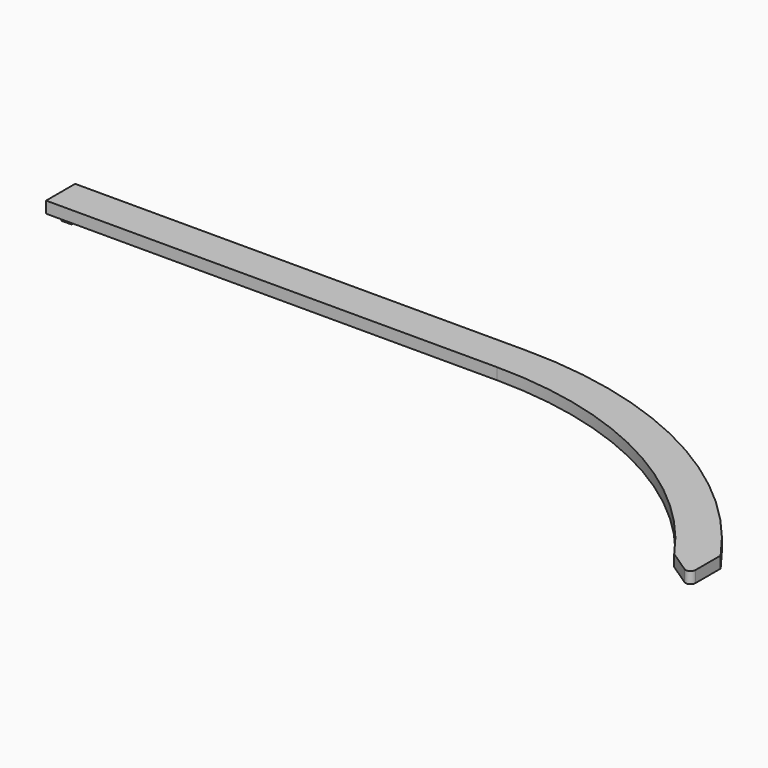
from build123d import *

# Parameters (mm, degrees)
F1_DEPTH = 2.3
F3_DEPTH = 2


with BuildPart() as f1:
    # F0 (on Top) → F1 (new body)
    with BuildSketch(Plane.XY):
        Polygon((45, 3.625), (-45, 3.625), (-45, 0), (-45, -3.625), (45, -3.625), align=None)
        Polygon((-44, -1), (-44, 0), (-44, 1), (-42, 1), (-42, -1), align=None, mode=Mode.SUBTRACT)
        with BuildLine():
            ThreePointArc((111.9139716029, -31.496938318), (82.7856789898, -5.6889854515), (45, 3.625))
            Line((45, 3.625), (45, -3.625))
            ThreePointArc((45, -3.625), (79.4162271285, -12.1084320129), (105.947070592, -35.615019464))
            Line((105.947070592, -35.615019464), (110.3610228539, -38.574432601))
            ThreePointArc((110.3610228539, -38.574432601), (111.3860089549, -38.6260052928), (111.9139716029, -37.7459418336))
            Line((111.9139716029, -37.7459418336), (111.9139716029, -31.496938318))
        make_face()
        Polygon((-44, 1), (-44, 0), (-44, -1), (-42, -1), (-42, 1), align=None)
    extrude(amount=-F1_DEPTH)

    # F2 (on face) → F3 (join)
    with BuildSketch(Plane(origin=(0, 0, -2.3), x_dir=(1, 0, 0), z_dir=(0, 0, -1))):
        Polygon((-44, 1), (-44, 0), (-44, -1), (-42, -1), (-42, 1), align=None)
    extrude(amount=F3_DEPTH)

    # F6 (on face) → F7 (revolve)
    with BuildSketch(Plane(origin=(0, 1, 0), x_dir=(-1, 0, 0), z_dir=(0, 1, 0))):
        with BuildLine():
            ThreePointArc((43.5, -3.3), (43.3535533906, -2.9464466094), (43, -2.8))
            Line((43, -2.8), (43, -3.3))
            Line((43, -3.3), (43.5, -3.3))
        make_face()
        with BuildLine():
            Line((43.5, -3.3), (43, -3.3))
            Line((43, -3.3), (43, -3.8))
            ThreePointArc((43, -3.8), (43.3535533906, -3.6535533906), (43.5, -3.3))
        make_face()
    revolve(axis=Axis((-43, 1, -3.3), (0, 0, -1)))


with BuildPart() as f5:
    # F4 (on face) → F5 (revolve)
    with BuildSketch(Plane.XZ.offset(1)):
        with BuildLine():
            Line((-43, -3.3), (-42.5, -3.3))
            ThreePointArc((-42.5, -3.3), (-42.6464466094, -2.9464466094), (-43, -2.8))
            Line((-43, -2.8), (-43, -3.3))
        make_face()
        with BuildLine():
            ThreePointArc((-43, -3.8), (-42.6464466094, -3.6535533906), (-42.5, -3.3))
            Line((-42.5, -3.3), (-43, -3.3))
            Line((-43, -3.3), (-43, -3.8))
        make_face()
    revolve(axis=Axis((-43, -1, -3.3), (0, 0, -1)))


solid = Compound([f1.part, f5.part])
